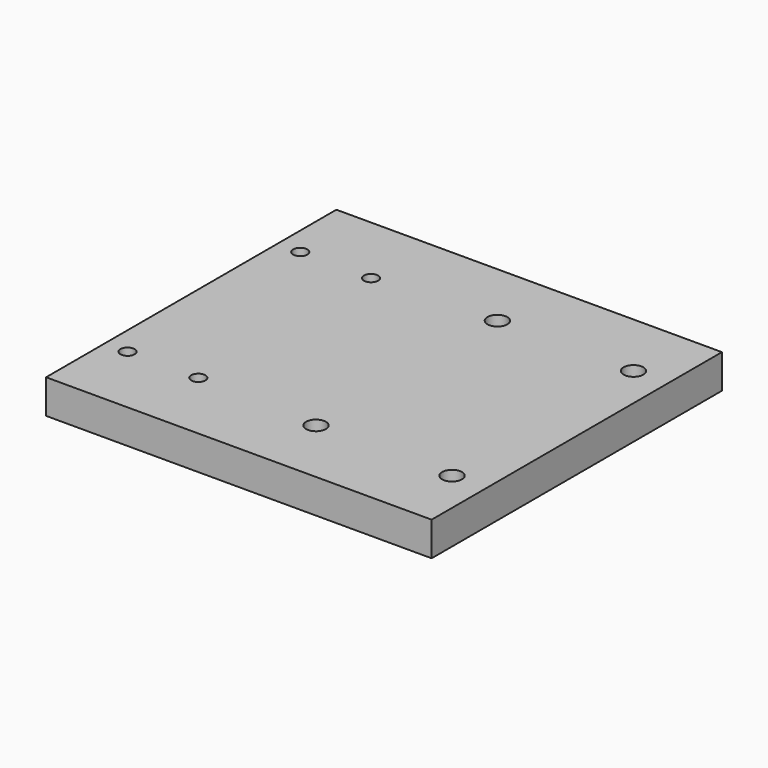
from build123d import *

# Parameters (mm, degrees)
F0_W     = 215.9
F0_H     = 203.2
F1_DEPTH = 19.05
F3_D     = 7.9375
F4_D     = 11.1125


# Not quite as in the source:
# - a length typed as a fraction of an inch, garbled in the dataset ("3 / 203.2 mm" for 3/8 in), is restored


with BuildPart() as f1:
    # F0 (on Top) → F1 (new body)
    with BuildSketch(Plane.XY):
        Rectangle(F0_W, F0_H)
    extrude(amount=F1_DEPTH)

    # F3 (through all)
    with Locations(Plane.XY.offset(19.05)):
        with Locations((-95.25, 60.452), (-55.626, 60.452), (-95.25, -60.452), (-55.626, -60.452)):
            Hole(F3_D / 2)

    # F4 (through all)
    with Locations(Plane.XY.offset(19.05)):
        with Locations((12.7, 63.5), (88.9, 63.5), (12.7, -63.5), (88.9, -63.5)):
            Hole(F4_D / 2)


solid = f1.part
